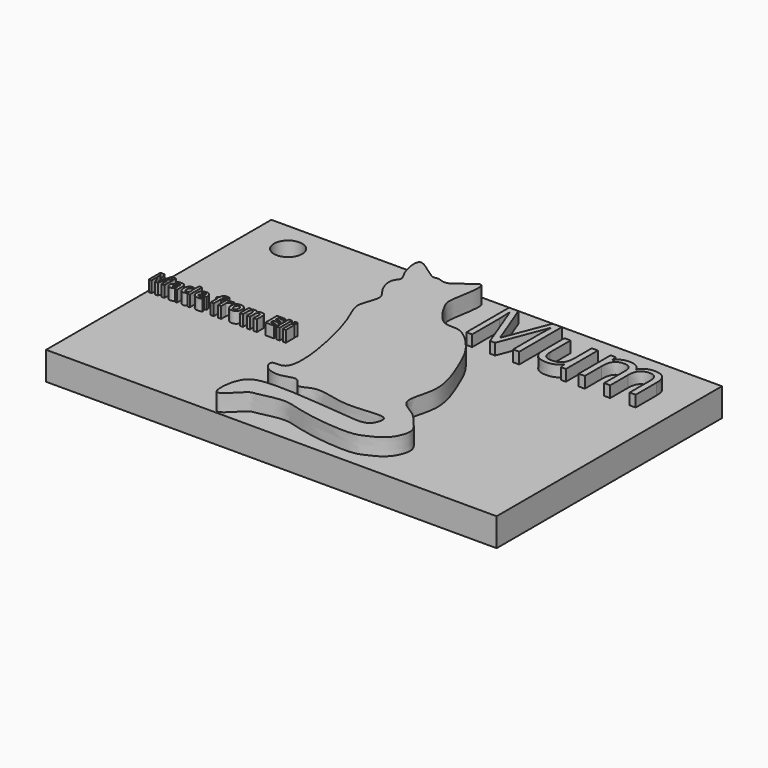
from build123d import *

# Parameters (mm, degrees)
F0_W         = 80
F0_H         = 50
F0_R         = 2.5
F1_DEPTH     = 5
F2_DEPTH     = 8
F3_TEXT_SIZE = 13.250771412
F4_DEPTH     = 2
F5_TEXT_SIZE = 3.6108871591
F6_DEPTH     = 2


# Not quite as in the source:
# - Text() gives the source's letters only with a copy of the font that has no kerning and outlines rounded to 1/6400 em; it was checked with that copy


with BuildPart() as f1:
    # F0 (on Top) → F1 (new body)
    with BuildSketch(Plane.XY):
        Rectangle(F0_W, F0_H)
        with Locations((-32.7451266348, 19.6470748633)):
            Circle(F0_R, mode=Mode.SUBTRACT)
        with BuildLine():
            add(Edge.make_bspline(
                [(1.6617914697, 11.3642968834), (2.5927244542, 10.8869494602), (4.7159151706, 11.7753096121), (9.1325248889, 7.1548353674), (10.7636726014, 3.5500128043), (13.5614184026, -3.1294501563), (12.8333488185, -7.1530823336), (11.6870086231, -10.9818503403), (15.3814029754, -12.5384148934), (16.9079839458, -14.7105725712), (18.6254352758, -16.3908757103), (18.195225816, -18.7270135496), (16.8824610658, -20.7868425609), (14.2751379389, -22.0745302746), (12.0068905883, -22.9676591856), (3.0411766949, -22.0854399512), (-0.8831656614, -20.268909455), (-5.3466965331, -21.7636362846), (-6.6113643886, -21.4533009002), (-10.8170974888, -26.9591970663), (-10.3371446471, -19.3274349316), (-6.5353150577, -17.3078667279), (7.8404359118, -18.9869159512), (12.0595852548, -19.2557169426), (13.1176644175, -17.7966665377), (13.5314992116, -15.1669411742), (5.9764380088, -17.1191001717), (0.2721717429, -14.3764251471), (-2.4670658259, -16.9501337122), (-3.5399344896, -13.9315190366), (-6.218362417, -15.6049459353), (-9.3460803948, -14.8070974972), (-10.0142360673, -12.3362001672), (-4.9760105282, -14.1569011089), (-8.8963526494, 4.2353700183), (-11.778805808, 7.6713332412), (-9.4102812468, 11.8501116593), (-11.5069871161, 13.5543206539), (-12.3751245184, 16.7792303808), (-10.8502483026, 17.9280684174), (-12.2474350851, 19.2701517786), (-13.5592584123, 25.7186669266), (-8.3241199397, 20.5067175062), (-7.2939478209, 21.4650856931), (-5.2889536933, 19.9026686649), (-0.0436518534, 26.3270791421), (-2.0791052269, 17.2319764681), (-1.8099218095, 15.6217249285), (0.4219425382, 12.0000447862), (1.6617914697, 11.3642968834)],
                knots=[0, 0, 0, 0, 0.0189451197, 0.0453821687, 0.0688996208, 0.0982386723, 0.121205307, 0.1414164158, 0.1619346167, 0.1804862003, 0.197027904, 0.2132854026, 0.2306845251, 0.2490155385, 0.2666950668, 0.299610058, 0.3239116586, 0.3464526616, 0.359826354, 0.3827104701, 0.4059298282, 0.4286092097, 0.4712438073, 0.4936014124, 0.5072722812, 0.5208577629, 0.5494109237, 0.5778069805, 0.5953040794, 0.6108525407, 0.6287395952, 0.648308086, 0.6615534327, 0.6780181995, 0.7226076518, 0.7478313457, 0.7689621326, 0.786286916, 0.8056918302, 0.8185279369, 0.8336821505, 0.8557221069, 0.8797262763, 0.8911934972, 0.9066256655, 0.9306805392, 0.9573038231, 0.9747682305, 1, 1, 1, 1], degree=3))
        make_face(mode=Mode.SUBTRACT)
    extrude(amount=F1_DEPTH)

    # F0 (on Top) → F2 (join)
    with BuildSketch(Plane.XY):
        with BuildLine():
            add(Edge.make_bspline(
                [(1.6617914697, 11.3642968834), (2.5927244542, 10.8869494602), (4.7159151706, 11.7753096121), (9.1325248889, 7.1548353674), (10.7636726014, 3.5500128043), (13.5614184026, -3.1294501563), (12.8333488185, -7.1530823336), (11.6870086231, -10.9818503403), (15.3814029754, -12.5384148934), (16.9079839458, -14.7105725712), (18.6254352758, -16.3908757103), (18.195225816, -18.7270135496), (16.8824610658, -20.7868425609), (14.2751379389, -22.0745302746), (12.0068905883, -22.9676591856), (3.0411766949, -22.0854399512), (-0.8831656614, -20.268909455), (-5.3466965331, -21.7636362846), (-6.6113643886, -21.4533009002), (-10.8170974888, -26.9591970663), (-10.3371446471, -19.3274349316), (-6.5353150577, -17.3078667279), (7.8404359118, -18.9869159512), (12.0595852548, -19.2557169426), (13.1176644175, -17.7966665377), (13.5314992116, -15.1669411742), (5.9764380088, -17.1191001717), (0.2721717429, -14.3764251471), (-2.4670658259, -16.9501337122), (-3.5399344896, -13.9315190366), (-6.218362417, -15.6049459353), (-9.3460803948, -14.8070974972), (-10.0142360673, -12.3362001672), (-4.9760105282, -14.1569011089), (-8.8963526494, 4.2353700183), (-11.778805808, 7.6713332412), (-9.4102812468, 11.8501116593), (-11.5069871161, 13.5543206539), (-12.3751245184, 16.7792303808), (-10.8502483026, 17.9280684174), (-12.2474350851, 19.2701517786), (-13.5592584123, 25.7186669266), (-8.3241199397, 20.5067175062), (-7.2939478209, 21.4650856931), (-5.2889536933, 19.9026686649), (-0.0436518534, 26.3270791421), (-2.0791052269, 17.2319764681), (-1.8099218095, 15.6217249285), (0.4219425382, 12.0000447862), (1.6617914697, 11.3642968834)],
                knots=[0, 0, 0, 0, 0.0189451197, 0.0453821687, 0.0688996208, 0.0982386723, 0.121205307, 0.1414164158, 0.1619346167, 0.1804862003, 0.197027904, 0.2132854026, 0.2306845251, 0.2490155385, 0.2666950668, 0.299610058, 0.3239116586, 0.3464526616, 0.359826354, 0.3827104701, 0.4059298282, 0.4286092097, 0.4712438073, 0.4936014124, 0.5072722812, 0.5208577629, 0.5494109237, 0.5778069805, 0.5953040794, 0.6108525407, 0.6287395952, 0.648308086, 0.6615534327, 0.6780181995, 0.7226076518, 0.7478313457, 0.7689621326, 0.786286916, 0.8056918302, 0.8185279369, 0.8336821505, 0.8557221069, 0.8797262763, 0.8911934972, 0.9066256655, 0.9306805392, 0.9573038231, 0.9747682305, 1, 1, 1, 1], degree=3))
        make_face()
    extrude(amount=F2_DEPTH)

    # F3 (on face) → F4 (join)
    with BuildSketch(Plane.XY.offset(5)):
        with Locations((3.3149365336, 12.5320857624)):
            Text('Mum', F3_TEXT_SIZE, font='Open Sans', text_align=(TextAlign.LEFT, TextAlign.BOTTOM))
    extrude(amount=F4_DEPTH)

    # F5 (on face) → F6 (join)
    with BuildSketch(Plane.XY.offset(5)):
        with Locations((-40, -2.5998387545)):
            Text('Made from Eli', F5_TEXT_SIZE, font='Open Sans', font_style=FontStyle.BOLD, text_align=(TextAlign.LEFT, TextAlign.BOTTOM))
    extrude(amount=F6_DEPTH)


solid = f1.part
